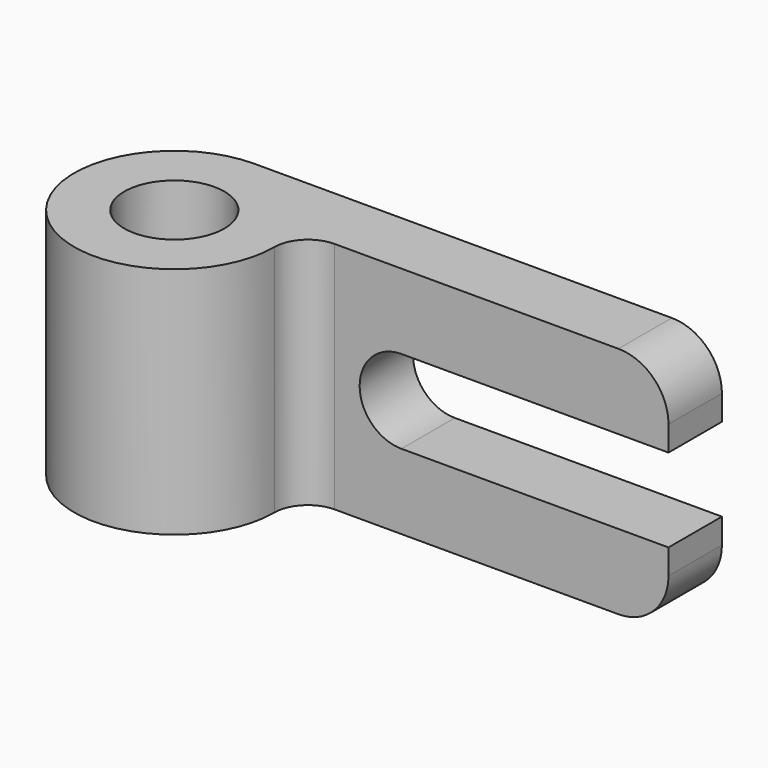
from build123d import *

# Parameters (mm, degrees)
F0_R        = 9.525
F1_DEPTH    = 44.45
F2_R        = 9.525
F3_T1_DEPTH = 44.45
F5_DEPTH    = 12.701


# Not quite as in the source:
# - a fillet or chamfer that OpenCascade refuses, or shapes differently, is made with other operations: its cross-section is extruded or revolved along the edge and cut away or added


with BuildPart() as f1:
    # F0 (on Top) → F1 (new body)
    with BuildSketch(Plane.XY):
        with BuildLine():
            Line((42.3913487732, -8.5454918444), (42.3913487732, 4.1545081556))
            Line((42.3913487732, 4.1545081556), (-46.5086512268, 4.1545081556))
            ThreePointArc((-46.5086512268, 4.1545081556), (-35.5101285987, 0.6587680223), (-28.5481389846, -8.5454918444))
            Line((-28.5481389846, -8.5454918444), (42.3913487732, -8.5454918444))
        make_face()
        with BuildLine():
            ThreePointArc((-28.5481389846, -8.5454918444), (-35.5101285987, 0.6587680223), (-46.5086512268, 4.1545081556))
            ThreePointArc((-46.5086512268, 4.1545081556), (-59.9790354084, -28.365876026), (-27.4586512268, -14.8954918444))
            ThreePointArc((-27.4586512268, -14.8954918444), (-27.7329986654, -11.6740991497), (-28.5481389846, -8.5454918444))
        make_face()
        with Locations((-46.5086512268, -14.8954918444)):
            Circle(F0_R, mode=Mode.SUBTRACT)
    extrude(amount=F1_DEPTH)

    # F2
    f2_edges = [f1.edges().sort_by_distance(p)[0] for p in [
        (42.391349, -2.195492, 44.45),
        (42.391349, -2.195492, 0),
    ]]
    fillet(f2_edges, radius=F2_R)

    # F3: fillet of radius 6.35 on 1 edges, made by hand

    # F3_s2 → F3_t1 (join)
    with BuildSketch(Plane.XY):
        with BuildLine():
            ThreePointArc((-21.1086512268, -8.5454918444), (-25.5987792873, -10.4053637839), (-27.4586512268, -14.8954918444))
            ThreePointArc((-27.4586512268, -14.8954918444), (-27.7329986654, -11.6740991497), (-28.5481389846, -8.5454918444))
            Line((-28.5481389846, -8.5454918444), (-21.1086512268, -8.5454918444))
        make_face()
    extrude(amount=F3_T1_DEPTH)

    # F4 (on face) → F5 (cut, through all)
    with BuildSketch(Plane.XZ.offset(8.5454918444)):
        with BuildLine():
            Line((42.3913487732, 14.2875), (42.3913487732, 30.1625))
            Line((42.3913487732, 30.1625), (-8.4086512268, 30.1625))
            ThreePointArc((-8.4086512268, 30.1625), (-16.3461512268, 22.225), (-8.4086512268, 14.2875))
            Line((-8.4086512268, 14.2875), (42.3913487732, 14.2875))
        make_face()
    extrude(amount=-F5_DEPTH, mode=Mode.SUBTRACT)


solid = f1.part
